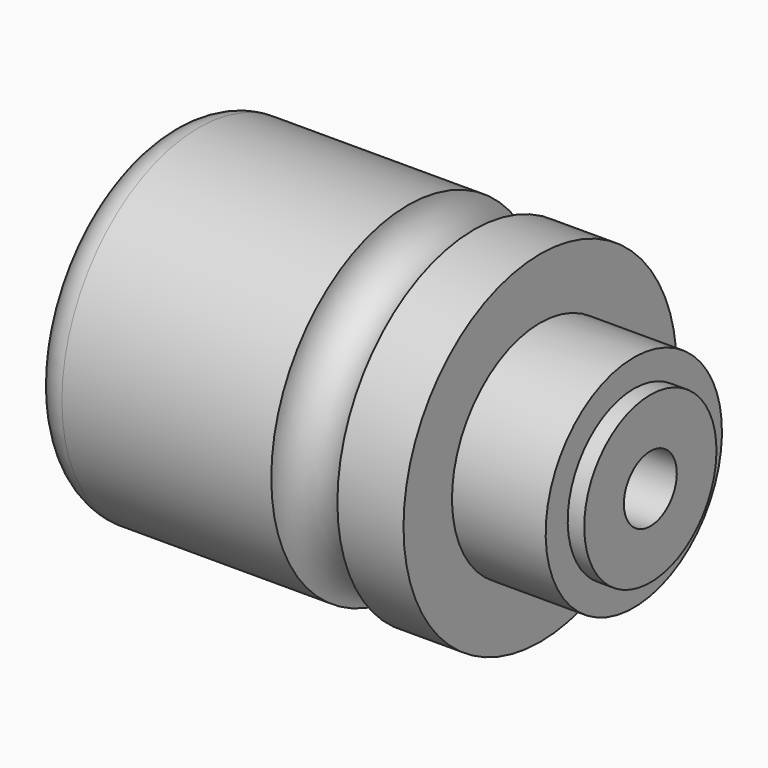
from build123d import *

# Parameters (mm, degrees)
F4_R = 5.99999


# Not quite as in the source:
# - a fillet or chamfer is up to 0.001 mm smaller than in the source, because OpenCascade refuses the exact size


with BuildPart() as f1:
    # F0 (on Front) → F1 (revolve)
    with BuildSketch(Plane.XZ):
        with BuildLine():
            Line((0, 31), (0, 0))
            Line((0, 0), (88, 0))
            Line((88, 0), (88, 15))
            Line((88, 15), (85, 15))
            Line((85, 15), (85, 20))
            Line((85, 20), (68, 20))
            Line((68, 20), (68, 31))
            Line((68, 31), (56, 31))
            ThreePointArc((56, 31), (50, 25), (44, 31))
            Line((44, 31), (0, 31))
        make_face()
    revolve(axis=Axis((44, 0, 0), (-1, 0, 0)))

    # F2 (on Front) → F3 (revolve, cut)
    with BuildSketch(Plane.XZ):
        Polygon((0, 25), (0, 0), (88, 0), (88, 6), (30, 6), (30, 16), (22, 16), (22, 20.5), (16.5, 20.5), (16.5, 12.5), (13.5, 12.5), (13.5, 16), (1.5, 16), (1.5, 25), align=None)
    revolve(axis=Axis((-10.2086656565, 0, 0), (-1, 0, 0)), mode=Mode.SUBTRACT)

    # F4 (radius 6 in the source; OpenCascade refuses exactly that, so slightly less here)
    f4_edges = [f1.edges().sort_by_distance(p)[0] for p in [
        (0, 0, -31),
    ]]
    fillet(f4_edges, radius=F4_R)


solid = f1.part
